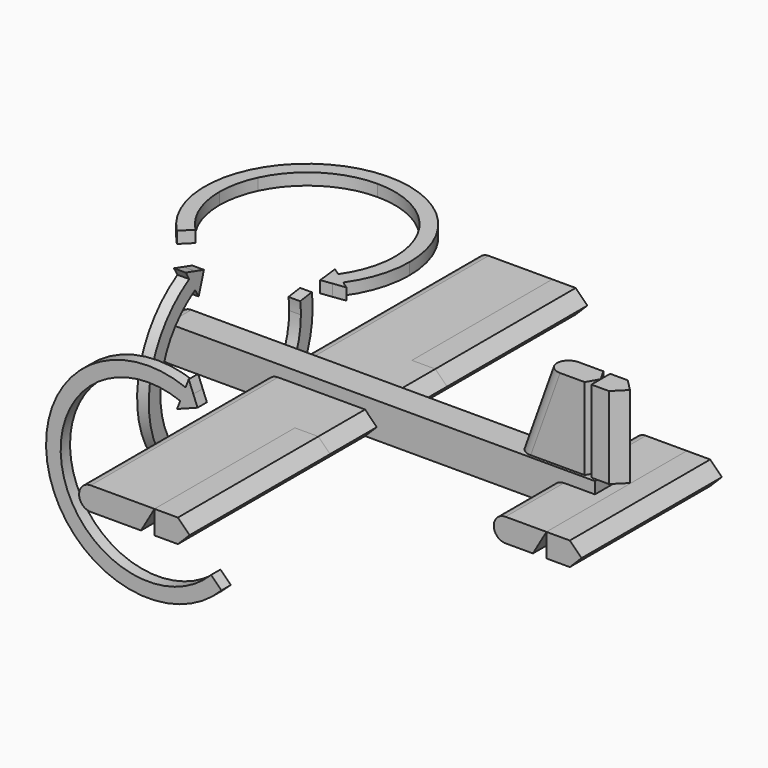
from build123d import *

# Parameters (mm, degrees)
F0_W        = 12.5
F0_H        = 4
F1_DEPTH    = 6
F2_DEPTH    = 4
F0_W_2      = 6
F0_H_2      = 30
F3_DEPTH    = 4
F4_DEPTH    = 20
F7_DEPTH    = 25
F8_DEPTH    = 5
F9_R        = 1.99999
F10_SIZE    = 1.99999
F10_2_SIZE  = 1.99999
F10_3_SIZE  = 1.99999
F10_4_SIZE  = 1.99999
F10_5_SIZE  = 1.99999
F11_SIZE2   = 2.309391
F11_SIZE    = 3.99999
F11_2_SIZE2 = 2.309391
F11_2_SIZE  = 3.99999
F11_3_SIZE2 = 2.309391
F11_3_SIZE  = 3.99999
F12_SIZE2   = 1.154691
F12_SIZE    = 1.99999
F15_DEPTH   = 2
F18_DEPTH   = 2
F21_DEPTH   = 2


# Not quite as in the source:
# - a fillet or chamfer is up to 0.001 mm smaller than in the source, because OpenCascade refuses the exact size


with BuildPart() as f1:
    # F0 (on Top) → F1 (new body)
    with BuildSketch(Plane.XY):
        Polygon((-58.7332326337, 24.4351043343), (-58.7332326337, 19.4351043343), (-39.9175214512, 19.4351043343), (-21.0230639726, 19.4351043343), (8.9769360274, 19.4351043343), (16.2667673663, 19.4351043343), (16.2667673663, 24.4351043343), (8.9769360274, 24.4351043343), (-21.0230639726, 24.4351043343), (-39.9175214512, 24.4351043343), align=None)
        with Locations((9.0167673663, 21.9351043343)):
            Rectangle(F0_W, F0_H, mode=Mode.SUBTRACT)
    extrude(amount=F1_DEPTH)

    # F0 (on Top) → F2 (join)
    with BuildSketch(Plane.XY):
        Polygon((-21.0230639726, 19.4351043343), (-39.9175214512, 19.4351043343), (-39.9175214512, -20.5648956657), (-27.0230639726, -20.5648956657), (-27.0230639726, 9.4351043343), (-21.0230639726, 9.4351043343), align=None)
        Polygon((-39.9175214512, 64.4351043343), (-39.9175214512, 24.4351043343), (-21.0230639726, 24.4351043343), (-21.0230639726, 34.4351043343), (-27.0230639726, 34.4351043343), (-27.0230639726, 64.4351043343), align=None)
        Polygon((16.2667673663, 19.4351043343), (8.9769360274, 19.4351043343), (8.9769360274, 6.9351043343), (17.9769360274, 6.9351043343), (17.9769360274, 36.9351043343), (8.9769360274, 36.9351043343), (8.9769360274, 24.4351043343), (16.2667673663, 24.4351043343), align=None)
    extrude(amount=F2_DEPTH)

    # F0 (on Top) → F4 (join)
    with BuildSketch(Plane.XY):
        with Locations((9.0167673663, 21.9351043343)):
            Rectangle(F0_W, F0_H)
    extrude(amount=F4_DEPTH)

    # F6 (on offset) → F7 (cut)
    with BuildSketch(Plane.XZ.offset(-19.9351043343)):
        Polygon((7.7822105959, 20), (2.7667673663, 20), (2.7667673663, 6), align=None)
    extrude(amount=-F7_DEPTH, mode=Mode.SUBTRACT)


with BuildPart() as f3:
    # F0 (on Top) → F3 (new body)
    with BuildSketch(Plane.XY):
        with Locations((-24.0230639726, -5.5648956657)):
            Rectangle(F0_W_2, F0_H_2)
    extrude(amount=F3_DEPTH)

    # F10#2 (size 2 in the source; OpenCascade refuses exactly that, so slightly less here)
    f10_2_edges = [f3.edges().sort_by_distance(p)[0] for p in [
        (-21.023064, -5.564896, 4),
        (-21.023064, -5.564896, 0),
    ]]
    chamfer(f10_2_edges, length=F10_2_SIZE)


with BuildPart() as f3b:
    # F0 (on Top) → F3, piece 2 (new body)
    with BuildSketch(Plane.XY):
        with Locations((-24.0230639726, 49.4351043343)):
            Rectangle(F0_W_2, F0_H_2)
    extrude(amount=F3_DEPTH)

    # F10#3 (size 2 in the source; OpenCascade refuses exactly that, so slightly less here)
    f10_3_edges = [f3b.edges().sort_by_distance(p)[0] for p in [
        (-21.023064, 49.435104, 4),
        (-21.023064, 49.435104, 0),
    ]]
    chamfer(f10_3_edges, length=F10_3_SIZE)


with BuildPart() as f3c:
    # F0 (on Top) → F3, piece 3 (new body)
    with BuildSketch(Plane.XY):
        with Locations((20.9769360274, 21.9351043343)):
            Rectangle(F0_W_2, F0_H_2)
    extrude(amount=F3_DEPTH)

    # F10#4 (size 2 in the source; OpenCascade refuses exactly that, so slightly less here)
    f10_4_edges = [f3c.edges().sort_by_distance(p)[0] for p in [
        (23.976936, 21.935104, 4),
        (23.976936, 21.935104, 0),
    ]]
    chamfer(f10_4_edges, length=F10_4_SIZE)


with BuildPart() as f8:
    # F8 (new): a face of the model
    f8_faces = [f1.part.faces().sort_by_distance(p)[0] for p in [
        (15.2667673663, 21.9351043343, 13),
    ]]
    extrude(f8_faces, amount=F8_DEPTH)

    # F10#5 (size 2 in the source; OpenCascade refuses exactly that, so slightly less here)
    f10_5_edges = [f8.edges().sort_by_distance(p)[0] for p in [
        (20.266767, 19.935104, 13),
        (20.266767, 23.935104, 13),
    ]]
    chamfer(f10_5_edges, length=F10_5_SIZE)


with BuildPart() as f1_1:
    add(f1.part)

    # F9 (radius 2 in the source; OpenCascade refuses exactly that, so slightly less here)
    f9_edges = [f1_1.edges().sort_by_distance(p)[0] for p in [
        (-39.917521, -0.564896, 4),
        (-39.917521, 44.435104, 4),
        (8.976936, 13.185104, 4),
        (-39.917521, -0.564896, 0),
        (-39.917521, 44.435104, 0),
        (8.976936, 13.185104, 0),
        (-58.733233, 21.935104, 6),
        (-58.733233, 21.935104, 0),
        (8.976936, 30.685104, 4),
        (8.976936, 30.685104, 0),
        (5.274489, 19.935104, 13),
        (5.274489, 23.935104, 13),
    ]]
    fillet(f9_edges, radius=F9_R)

    # F10 (size 2 in the source; OpenCascade refuses exactly that, so slightly less here)
    f10_edges = [f1_1.edges().sort_by_distance(p)[0] for p in [
        (-21.023064, 14.435104, 4),
        (-21.023064, 29.435104, 4),
        (-21.023064, 14.435104, 0),
        (-21.023064, 29.435104, 0),
    ]]
    chamfer(f10_edges, length=F10_SIZE)

    # F11 (size 4 and 2.3094010768 in the source; OpenCascade refuses exactly that, so slightly less here)
    f11_edges = [f1_1.edges().sort_by_distance(p)[0] for p in [
        (-27.023064, -5.564896, 0),
    ]]
    f11_side = f1_1.faces().sort_by_distance((-27.023064, -5.564896, 2))[0]
    chamfer(f11_edges, length=F11_SIZE, length2=F11_SIZE2, reference=f11_side)

    # F11#2 (size 4 and 2.3094010768 in the source; OpenCascade refuses exactly that, so slightly less here)
    f11_2_edges = [f1_1.edges().sort_by_distance(p)[0] for p in [
        (-27.023064, 49.435104, 0),
    ]]
    f11_2_side = f1_1.faces().sort_by_distance((-27.023064, 49.435104, 2))[0]
    chamfer(f11_2_edges, length=F11_2_SIZE, length2=F11_2_SIZE2, reference=f11_2_side)

    # F11#3 (size 4 and 2.3094010768 in the source; OpenCascade refuses exactly that, so slightly less here)
    f11_3_edges = [f1_1.edges().sort_by_distance(p)[0] for p in [
        (17.976936, 21.935104, 0),
    ]]
    f11_3_side = f1_1.faces().sort_by_distance((17.976936, 21.935104, 2))[0]
    chamfer(f11_3_edges, length=F11_3_SIZE, length2=F11_3_SIZE2, reference=f11_3_side)

    # F12 (size 2 and 1.1547005384 in the source; OpenCascade refuses exactly that, so slightly less here)
    f12_edges = [f1_1.edges().sort_by_distance(p)[0] for p in [
        (15.266767, 19.935104, 13),
        (15.266767, 23.935104, 13),
    ]]
    f12_side = f1_1.faces().sort_by_distance((15.266767, 21.935104, 13))[0]
    chamfer(f12_edges, length=F12_SIZE, length2=F12_SIZE2, reference=f12_side)


with BuildPart() as f15:
    # F14 (on offset) → F15 (new body)
    with BuildSketch(Plane.YZ.offset(-50)):
        with BuildLine():
            Line((30.5101656349, -12.2551081179), (29.2851568777, -10.0758069582))
            ThreePointArc((29.2851568777, -10.0758069582), (8.9307815246, -4.4758001753), (14.3342516917, 15.9316294065))
            Line((14.3342516917, 15.9316294065), (13.0674429179, 18.0869009742))
            ThreePointArc((13.0674429179, 18.0869009742), (6.7633943897, -5.7217668712), (30.5101656349, -12.2551081179))
        make_face()
        with BuildLine():
            ThreePointArc((14.3342516917, 15.9316294065), (15.0210934818, 16.311515839), (15.7268663052, 16.6549544333))
            Line((15.7268663052, 16.6549544333), (16.2145903627, 18.2098067016))
            Line((16.2145903627, 18.2098067016), (14.3468390864, 18.769217816))
            ThreePointArc((14.3468390864, 18.769217816), (13.7000712643, 18.4413156932), (13.0674429179, 18.0869009742))
            Line((13.0674429179, 18.0869009742), (14.3342516917, 15.9316294065))
        make_face()
        with BuildLine():
            Line((14.3342516917, 15.9316294065), (15.094336956, 14.6384664658))
            Line((15.094336956, 14.6384664658), (15.7268663052, 16.6549544333))
            ThreePointArc((15.7268663052, 16.6549544333), (15.0210934818, 16.311515839), (14.3342516917, 15.9316294065))
        make_face()
        with BuildLine():
            ThreePointArc((13.0674429179, 18.0869009742), (13.7000712643, 18.4413156932), (14.3468390864, 18.769217816))
            Line((14.3468390864, 18.769217816), (12.3073576537, 19.3800639148))
            Line((12.3073576537, 19.3800639148), (13.0674429179, 18.0869009742))
        make_face()
        with BuildLine():
            Line((39.259186316, 5.4751128239), (36.7843174615, 5.1215252776))
            ThreePointArc((36.7843174615, 5.1215252776), (36.8973601286, 4.0634385484), (36.9351043343, 3))
            ThreePointArc((36.9351043343, 3), (34.8821269293, -4.5746026909), (29.2851568777, -10.0758069582))
            Line((29.2851568777, -10.0758069582), (30.5101656349, -12.2551081179))
            ThreePointArc((30.5101656349, -12.2551081179), (37.0399640285, -5.8370364727), (39.4351043343, 3))
            ThreePointArc((39.4351043343, 3), (39.3910694276, 4.2406783064), (39.259186316, 5.4751128239))
        make_face()
    extrude(amount=F15_DEPTH)


with BuildPart() as f18:
    # F17 (on offset) → F18 (new body)
    with BuildSketch(Plane.XZ.offset(10)):
        with BuildLine():
            Line((-22.4187029305, -10.2486544399), (-24.2042484335, -8.4988466628))
            ThreePointArc((-24.2042484335, -8.4988466628), (-49.5813990611, -1.1576404862), (-29.4749108405, 15.9777676952))
            Line((-29.4749108405, 15.9777676952), (-28.5678090721, 18.3073956444))
            ThreePointArc((-28.5678090721, 18.3073956444), (-52.0253786628, -1.6839139005), (-22.4187029305, -10.2486544399))
        make_face()
        with BuildLine():
            Line((-28.5678090721, 18.3073956444), (-29.4749108405, 15.9777676952))
            ThreePointArc((-29.4749108405, 15.9777676952), (-28.751203924, 15.6739360886), (-28.0443808054, 15.3326643123))
            Line((-28.0443808054, 15.3326643123), (-26.5216797206, 15.9130277666))
            Line((-26.5216797206, 15.9130277666), (-27.2396089112, 17.7257641795))
            ThreePointArc((-27.2396089112, 17.7257641795), (-27.8976824924, 18.0303418863), (-28.5678090721, 18.3073956444))
        make_face()
        with BuildLine():
            ThreePointArc((-28.0443808054, 15.3326643123), (-28.751203924, 15.6739360886), (-29.4749108405, 15.9777676952))
            Line((-29.4749108405, 15.9777676952), (-30.0191719016, 14.5799909257))
            Line((-30.0191719016, 14.5799909257), (-28.0443808054, 15.3326643123))
        make_face()
        with BuildLine():
            Line((-28.023548011, 19.7051724139), (-28.5678090721, 18.3073956444))
            ThreePointArc((-28.5678090721, 18.3073956444), (-27.8976824924, 18.0303418863), (-27.2396089112, 17.7257641795))
            Line((-27.2396089112, 17.7257641795), (-28.023548011, 19.7051724139))
        make_face()
    extrude(amount=F18_DEPTH)


with BuildPart() as f21:
    # F20 (on offset) → F21 (new body)
    with BuildSketch(Plane.XY.offset(25)):
        with BuildLine():
            ThreePointArc((-34.9175214512, 39.4351043343), (-44.2654551052, 36.729229398), (-50.7226071157, 29.4483770657))
            Line((-50.7226071157, 29.4483770657), (-48.4647377351, 28.3750523898))
            ThreePointArc((-48.4647377351, 28.3750523898), (-42.9300360118, 34.6157829603), (-34.9175214512, 36.9351043343))
            Line((-34.9175214512, 36.9351043343), (-34.9175214512, 39.4351043343))
        make_face()
        with BuildLine():
            Line((-22.686037665, 13.2523165108), (-23.9091860436, 14.1205952931))
            Line((-23.9091860436, 14.1205952931), (-23.6600991667, 12.0219593484))
            ThreePointArc((-23.6600991667, 12.0219593484), (-23.1569678169, 12.6243912459), (-22.686037665, 13.2523165108))
        make_face()
        with BuildLine():
            Line((-23.4680358856, 10.4037652844), (-21.5350369428, 10.6586195813))
            ThreePointArc((-21.5350369428, 10.6586195813), (-21.0793669968, 11.2227058495), (-20.6474570339, 11.8051852068))
            Line((-20.6474570339, 11.8051852068), (-22.686037665, 13.2523165108))
            ThreePointArc((-22.686037665, 13.2523165108), (-23.1569678169, 12.6243912459), (-23.6600991667, 12.0219593484))
            Line((-23.6600991667, 12.0219593484), (-23.4680358856, 10.4037652844))
        make_face()
        with BuildLine():
            ThreePointArc((-20.6474570339, 11.8051852068), (-21.0793669968, 11.2227058495), (-21.5350369428, 10.6586195813))
            Line((-21.5350369428, 10.6586195813), (-19.4243086553, 10.9369064245))
            Line((-19.4243086553, 10.9369064245), (-20.6474570339, 11.8051852068))
        make_face()
        with BuildLine():
            ThreePointArc((-50.7226071157, 29.4483770657), (-52.168080783, 18.9909231681), (-47.3358865818, 9.6048891098))
            Line((-47.3358865818, 9.6048891098), (-45.5618344203, 11.3663484276))
            ThreePointArc((-45.5618344203, 11.3663484276), (-48.7859152755, 16.2195420057), (-49.9175214512, 21.9351043343))
            ThreePointArc((-49.9175214512, 21.9351043343), (-49.5498186778, 25.2359948006), (-48.4647377351, 28.3750523898))
            Line((-48.4647377351, 28.3750523898), (-50.7226071157, 29.4483770657))
        make_face()
        with BuildLine():
            Line((-34.9175214512, 39.4351043343), (-34.9175214512, 36.9351043343))
            ThreePointArc((-34.9175214512, 36.9351043343), (-24.3109197334, 32.5417060521), (-19.9175214512, 21.9351043343))
            ThreePointArc((-19.9175214512, 21.9351043343), (-20.6264008374, 17.3783651928), (-22.686037665, 13.2523165108))
            Line((-22.686037665, 13.2523165108), (-20.6474570339, 11.8051852068))
            ThreePointArc((-20.6474570339, 11.8051852068), (-18.2445474018, 16.6189086692), (-17.4175214512, 21.9351043343))
            ThreePointArc((-17.4175214512, 21.9351043343), (-22.5431527804, 34.309473005), (-34.9175214512, 39.4351043343))
        make_face()
    extrude(amount=F21_DEPTH)


solid = Compound([f3.part, f3b.part, f3c.part, f8.part, f1_1.part, f15.part, f18.part, f21.part])
